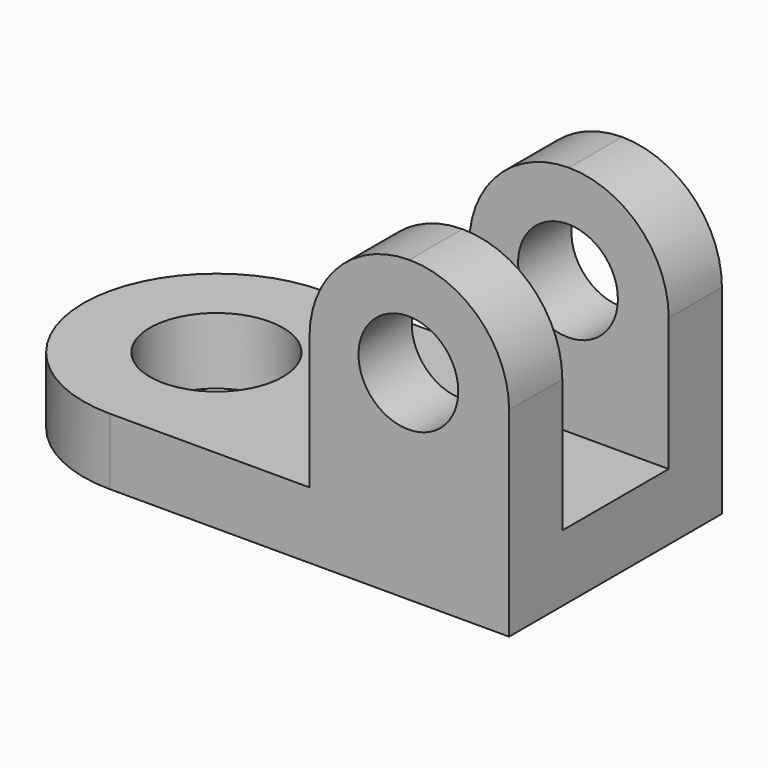
from build123d import *

# Parameters (mm, degrees)
F0_W      = 101.6
F0_H      = 50.8
F1_DEPTH  = 12.7
F2_R      = 25.39999
F3_R      = 12.7
F4_DEPTH  = 12.701
F5_W      = 38.1
F5_H      = 12.7
F6_DEPTH  = 44.45
F7_R      = 19.04999
F8_W      = 38.1
F8_H      = 12.7
F9_DEPTH  = 44.45
F10_R     = 19.04999
F11_R     = 9.525
F12_DEPTH = 50.801


# Not quite as in the source:
# - a fillet or chamfer is up to 0.001 mm smaller than in the source, because OpenCascade refuses the exact size


with BuildPart() as f1:
    # F0 (on Top) → F1 (new body)
    with BuildSketch(Plane.XY):
        with Locations((2.7364386797, -9.4244979978)):
            Rectangle(F0_W, F0_H)
    extrude(amount=F1_DEPTH)

    # F2 (radius 25.4 in the source; OpenCascade refuses exactly that, so slightly less here)
    f2_edges = [f1.edges().sort_by_distance(p)[0] for p in [
        (-48.063561, 15.975502, 6.35),
        (-48.063561, -34.824498, 6.35),
    ]]
    fillet(f2_edges, radius=F2_R)

    # F3 (on face) → F4 (cut, through all)
    with BuildSketch(Plane.XY.offset(12.7)):
        with Locations((-22.6635613203, -9.4244979978)):
            Circle(F3_R)
    extrude(amount=-F4_DEPTH, mode=Mode.SUBTRACT)

    # F5 (on face) → F6 (join)
    with BuildSketch(Plane.XY.offset(12.7)):
        with Locations((34.4864386797, -28.4744979978)):
            Rectangle(F5_W, F5_H)
    extrude(amount=F6_DEPTH)

    # F7 (radius 19.05 in the source; OpenCascade refuses exactly that, so slightly less here)
    f7_edges = [f1.edges().sort_by_distance(p)[0] for p in [
        (15.436439, -28.474498, 57.15),
        (53.536439, -28.474498, 57.15),
    ]]
    fillet(f7_edges, radius=F7_R)

    # F8 (on face) → F9 (join)
    with BuildSketch(Plane.XY.offset(12.7)):
        with Locations((34.4864386797, 9.6255020022)):
            Rectangle(F8_W, F8_H)
    extrude(amount=F9_DEPTH)

    # F10 (radius 19.05 in the source; OpenCascade refuses exactly that, so slightly less here)
    f10_edges = [f1.edges().sort_by_distance(p)[0] for p in [
        (15.436439, 9.625502, 57.15),
        (53.536439, 9.625502, 57.15),
    ]]
    fillet(f10_edges, radius=F10_R)

    # F11 (on face) → F12 (cut, through all)
    with BuildSketch(Plane.XZ.offset(34.8244979978)):
        with Locations((34.3096069992, 38.1)):
            Circle(F11_R)
    extrude(amount=-F12_DEPTH, mode=Mode.SUBTRACT)


solid = f1.part
